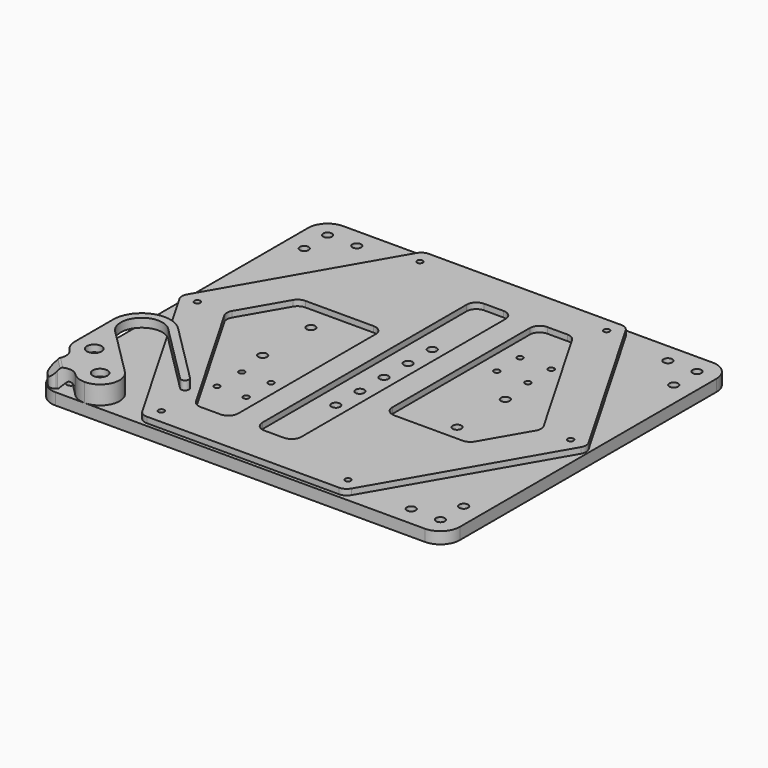
from build123d import *

# Parameters (mm, degrees)
F0_W          = 210
F0_H          = 185
F0_R          = 2
F1_DEPTH      = 6
F2_R          = 10
F3_R          = 1.5
F4_DEPTH      = 6.001
F5_R          = 2.25
F6_DEPTH      = 6.001
F7_R          = 2.25
F8_DEPTH      = 6.001
F9_R          = 2.25
F10_DEPTH     = 6.001
F11_R         = 1.5
F12_DEPTH     = 3
F13_W         = 12.5
F13_H         = 141.2768775266
F14_DEPTH     = 3
F16_DEPTH     = 3
F17_R         = 5
F18_R         = 1.5
F19_DEPTH     = 5
F20_R         = 1.5
F21_DEPTH     = 4.5
F22_R         = 3.75
F23_DEPTH     = 3.5
F24_SIZE      = 2.24999
F26_DEPTH     = 9.5
F28_DEPTH     = 9.5
F29_SIZE      = 5
F31_DEPTH     = 8
F32_T4_DEPTH  = 19.75
F32_T11_DEPTH = 19.75
F33_R         = 3
F34_R         = 1.5


# Not quite as in the source:
# - a fillet or chamfer that OpenCascade refuses, or shapes differently, is made with other operations: its cross-section is extruded or revolved along the edge and cut away or added
# - a fillet or chamfer is up to 0.001 mm smaller than in the source, because OpenCascade refuses the exact size


with BuildPart() as f1:
    # F0 (on Top) → F1 (new body)
    with BuildSketch(Plane.XY):
        Rectangle(F0_W, F0_H)
        with Locations((-48, -83.1384387633)):
            Circle(F0_R, mode=Mode.SUBTRACT)
        with Locations((48, -83.1384387633)):
            Circle(F0_R, mode=Mode.SUBTRACT)
        with Locations((-96, 0)):
            Circle(F0_R, mode=Mode.SUBTRACT)
        with Locations((-48, 83.1384387633)):
            Circle(F0_R, mode=Mode.SUBTRACT)
        with Locations((96, 0)):
            Circle(F0_R, mode=Mode.SUBTRACT)
        with Locations((48, 83.1384387633)):
            Circle(F0_R, mode=Mode.SUBTRACT)
    extrude(amount=F1_DEPTH)

    # F2
    f2_edges = [f1.edges().sort_by_distance(p)[0] for p in [
        (-105, -92.5, 3),
        (105, -92.5, 3),
        (-105, 92.5, 3),
        (105, 92.5, 3),
    ]]
    fillet(f2_edges, radius=F2_R)

    # F3 (on face) → F4 (cut, through all)
    with BuildSketch(Plane(origin=(0, 0, 0), x_dir=(1, 0, 0), z_dir=(0, 0, -1))):
        with Locations((-47.5, 48)):
            Circle(F3_R)
        with Locations((-32.5, 48)):
            Circle(F3_R)
        with Locations((-47.5, 32)):
            Circle(F3_R)
        with Locations((-32.5, 32)):
            Circle(F3_R)
        with Locations((32, -47.5)):
            Circle(F3_R)
        with Locations((32, -32.5)):
            Circle(F3_R)
        with Locations((48, -32.5)):
            Circle(F3_R)
        with Locations((48, -47.5)):
            Circle(F3_R)
    extrude(amount=-F4_DEPTH, mode=Mode.SUBTRACT)

    # F5 (on face) → F6 (cut, through all)
    with BuildSketch(Plane(origin=(0, 0, 0), x_dir=(1, 0, 0), z_dir=(0, 0, -1))):
        with Locations((0, -31)):
            Circle(F5_R)
        Circle(F5_R)
        with Locations((0, 31)):
            Circle(F5_R)
        with Locations((0, -15.5)):
            Circle(F5_R)
        with Locations((0, 15.5)):
            Circle(F5_R)
    extrude(amount=-F6_DEPTH, mode=Mode.SUBTRACT)

    # F7 (on face) → F8 (cut, through all)
    with BuildSketch(Plane(origin=(0, 0, 0), x_dir=(1, 0, 0), z_dir=(0, 0, -1))):
        with Locations((50, 15.5)):
            Circle(F7_R)
        with Locations((50, -15.5)):
            Circle(F7_R)
        with Locations((-50, 15.5)):
            Circle(F7_R)
        with Locations((-50, -15.5)):
            Circle(F7_R)
    extrude(amount=-F8_DEPTH, mode=Mode.SUBTRACT)

    # F9 (on face) → F10 (cut, through all)
    with BuildSketch(Plane(origin=(0, 0, 0), x_dir=(1, 0, 0), z_dir=(0, 0, -1))):
        with Locations((95, 82.5)):
            Circle(F9_R)
        with Locations((95, 67.5)):
            Circle(F9_R)
        with Locations((80, 82.5)):
            Circle(F9_R)
        with Locations((-95, 67.5)):
            Circle(F9_R)
        with Locations((-95, 82.5)):
            Circle(F9_R)
        with Locations((-80, 82.5)):
            Circle(F9_R)
        with Locations((95, -67.5)):
            Circle(F9_R)
        with Locations((95, -82.5)):
            Circle(F9_R)
        with Locations((80, -82.5)):
            Circle(F9_R)
        with Locations((-95, -67.5)):
            Circle(F9_R)
        with Locations((-95, -82.5)):
            Circle(F9_R)
        with Locations((-80, -82.5)):
            Circle(F9_R)
    extrude(amount=-F10_DEPTH, mode=Mode.SUBTRACT)


with BuildPart() as f12:
    # F11 (on face) → F12 (new body)
    with BuildSketch(Plane.XY.offset(6)):
        Polygon((52.3301270189, -90.6384387633), (104.6602540378, 0), (52.3301270189, 90.6384387633), (-52.3301270189, 90.6384387633), (-104.6602540378, 0), (-52.3301270189, -90.6384387633), align=None)
        with Locations((-48, -83.1384387633)):
            Circle(F11_R, mode=Mode.SUBTRACT)
        with Locations((48, -83.1384387633)):
            Circle(F11_R, mode=Mode.SUBTRACT)
        with Locations((-96, 0)):
            Circle(F11_R, mode=Mode.SUBTRACT)
        with Locations((-48, 83.1384387633)):
            Circle(F11_R, mode=Mode.SUBTRACT)
        Polygon((40.7831216351, 70.6384387633), (81.5662432703, 0), (40.7831216351, -70.6384387633), (-40.7831216351, -70.6384387633), (-81.5662432703, 0), (-40.7831216351, 70.6384387633), align=None, mode=Mode.SUBTRACT)
        with Locations((96, 0)):
            Circle(F11_R, mode=Mode.SUBTRACT)
        with Locations((48, 83.1384387633)):
            Circle(F11_R, mode=Mode.SUBTRACT)
    extrude(amount=F12_DEPTH)

    # F13 (on face) → F14 (join, through all)
    with BuildSketch(Plane.XY.offset(9)):
        with Locations((-16.25, 0)):
            Rectangle(F13_W, F13_H)
        with Locations((16.25, 0)):
            Rectangle(F13_W, F13_H)
    extrude(amount=-F14_DEPTH)

    # F15 (on face) → F16 (join, through all)
    with BuildSketch(Plane.XY.offset(9)):
        Polygon((-22.5, 70.6384387633), (-40.7831216351, 70.6384387633), (-65.5447733002, 27.75), (-22.5, 27.75), align=None)
        Polygon((22.5, -27.75), (22.5, -70.6384387633), (40.7831216351, -70.6384387633), (65.5447733002, -27.75), align=None)
    extrude(amount=-F16_DEPTH)

    # F17
    f17_edges = [f12.edges().sort_by_distance(p)[0] for p in [
        (-52.330127, 90.638439, 7.5),
        (-104.660254, 0, 7.5),
        (-52.330127, -90.638439, 7.5),
        (52.330127, -90.638439, 7.5),
        (104.660254, 0, 7.5),
        (52.330127, 90.638439, 7.5),
        (-81.566243, 0, 7.5),
        (-40.783122, -70.638439, 7.5),
        (-22.5, -70.638439, 7.5),
        (-65.544773, 27.75, 7.5),
        (-22.5, 27.75, 7.5),
        (-10, 70.638439, 7.5),
        (10, 70.638439, 7.5),
        (10, -70.638439, 7.5),
        (-10, -70.638439, 7.5),
        (22.5, -27.75, 7.5),
        (65.544773, -27.75, 7.5),
        (81.566243, 0, 7.5),
        (40.783122, 70.638439, 7.5),
        (22.5, 70.638439, 7.5),
    ]]
    fillet(f17_edges, radius=F17_R)


with BuildPart() as f19:
    # F18 (on face) → F19 (new body)
    with BuildSketch(Plane.XY.offset(6)):
        with BuildLine():
            Line((-105, -67.5), (-105, -82.5))
            ThreePointArc((-105, -82.5), (-102.0710678119, -89.5710678119), (-95, -92.5))
            Line((-95, -92.5), (-80, -92.5))
            ThreePointArc((-80, -92.5), (-70.7612046749, -86.3268343237), (-72.9289321881, -75.4289321881))
            Line((-72.9289321881, -75.4289321881), (-87.9289321881, -60.4289321881))
            ThreePointArc((-87.9289321881, -60.4289321881), (-98.8268343237, -58.2612046749), (-105, -67.5))
        make_face()
        with Locations((-95, -82.5)):
            Circle(F18_R, mode=Mode.SUBTRACT)
        with Locations((-80, -82.5)):
            Circle(F18_R, mode=Mode.SUBTRACT)
        with Locations((-95, -67.5)):
            Circle(F18_R, mode=Mode.SUBTRACT)
    extrude(amount=F19_DEPTH)

    # F20 (on face) → F21 (join)
    with BuildSketch(Plane.XY.offset(11)):
        with BuildLine():
            Line((-72.9289321881, -75.4289321881), (-87.9289321881, -60.4289321881))
            Line((-87.9289321881, -60.4289321881), (-97.8653320081, -50.4925323681))
            ThreePointArc((-97.8653320081, -50.4925323681), (-97.8653320081, -35.3570164091), (-82.7298160491, -35.3570164091))
            Line((-82.7298160491, -35.3570164091), (-51.9723484172, -66.1144840409))
            ThreePointArc((-51.9723484172, -66.1144840409), (-49.1439212925, -66.1144840409), (-49.1439212925, -63.2860569162))
            Line((-49.1439212925, -63.2860569162), (-79.9013889243, -32.5285892843))
            ThreePointArc((-79.9013889243, -32.5285892843), (-95.9239488634, -29.3415039554), (-105, -42.9247743886))
            Line((-105, -42.9247743886), (-105, -67.5))
            Line((-105, -67.5), (-105, -82.5))
            ThreePointArc((-105, -82.5), (-102.0710678119, -89.5710678119), (-95, -92.5))
            Line((-95, -92.5), (-80, -92.5))
            ThreePointArc((-80, -92.5), (-70.7612046749, -86.3268343237), (-72.9289321881, -75.4289321881))
        make_face()
        with Locations((-95, -82.5)):
            Circle(F20_R, mode=Mode.SUBTRACT)
        with Locations((-80, -82.5)):
            Circle(F20_R, mode=Mode.SUBTRACT)
        with Locations((-95, -67.5)):
            Circle(F20_R, mode=Mode.SUBTRACT)
    extrude(amount=F21_DEPTH)

    # F22 (on face) → F23 (cut)
    with BuildSketch(Plane.XY.offset(15.5)):
        with Locations((-95, -67.5)):
            Circle(F22_R)
        with Locations((-80, -82.5)):
            Circle(F22_R)
    extrude(amount=-F23_DEPTH, mode=Mode.SUBTRACT)

    # F24 (size 2.25 in the source; OpenCascade refuses exactly that, so slightly less here)
    f24_edges = [f19.edges().sort_by_distance(p)[0] for p in [
        (-96.5, -67.5, 12),
        (-81.5, -82.5, 12),
    ]]
    chamfer(f24_edges, length=F24_SIZE)

    # F25 (on face) → F26 (cut, through all)
    with BuildSketch(Plane.XY.offset(15.5)):
        with BuildLine():
            ThreePointArc((-102.0710678119, -74.5710678119), (-104.2387953251, -71.3268343237), (-105, -67.5))
            Line((-105, -67.5), (-105, -82.5))
            ThreePointArc((-105, -82.5), (-102.0710678119, -89.5710678119), (-95, -92.5))
            Line((-95, -92.5), (-80, -92.5))
            ThreePointArc((-80, -92.5), (-83.8268343237, -91.7387953251), (-87.0710678119, -89.5710678119))
            Line((-87.0710678119, -89.5710678119), (-102.0710678119, -74.5710678119))
        make_face()
    extrude(amount=-F26_DEPTH, mode=Mode.SUBTRACT)

    # F27 (on face) → F28 (join, through all)
    with BuildSketch(Plane.XY.offset(15.5)):
        Polygon((-89.6213203436, -82.7781745931), (-95.2781745931, -77.1213203436), (-104.4705627485, -86.313708499), (-98.813708499, -91.9705627485), align=None)
    extrude(amount=-F28_DEPTH)

    # F29
    f29_edges = [f19.edges().sort_by_distance(p)[0] for p in [
        (-101.642136, -89.142136, 15.5),
    ]]
    chamfer(f29_edges, length=F29_SIZE)

    # F30 (on face) → F31 (cut, through all)
    with BuildSketch(Plane(origin=(-3.4215728753, 3.4215728753, 0), x_dir=(0.7071067812, 0.7071067812, 0), z_dir=(0.7071067812, -0.7071067812, 0))):
        Polygon((-124.9048519428, 6), (-124.9048519428, 12), (-130.9048519428, 6), align=None)
    extrude(amount=-F31_DEPTH, mode=Mode.SUBTRACT)

    # F32: fillet of radius 6.5 on 2 edges, made by hand


with BuildPart() as f32_tool2:
    # F32_s3 → F32_t4 (new body)
    with BuildSketch(Plane.XY.offset(15.5)):
        with BuildLine():
            ThreePointArc((-96.3388347648, -89.4956890143), (-91.7426406871, -87.591883092), (-87.1464466094, -89.4956890143))
            Line((-87.1464466094, -89.4956890143), (-91.7426406871, -84.8994949366))
            Line((-91.7426406871, -84.8994949366), (-96.3388347648, -89.4956890143))
        make_face()
    extrude(amount=-F32_T4_DEPTH)

    split(bisect_by=Plane.XY.offset(6), keep=Keep.TOP)

    split(bisect_by=Plane(origin=(-48.4031745931, -48.4031745931, 68.4524259714), x_dir=(0.7071067812, -0.7071067812, 0), z_dir=(-0.5, -0.5, 0.7071067812)), keep=Keep.TOP)

    split(bisect_by=Plane(origin=(-51.4083784131, -51.4083784131, 72.7024259714), x_dir=(-0.7071067812, 0.7071067812, 0), z_dir=(0.5, 0.5, -0.7071067812)), keep=Keep.TOP)


with BuildPart() as f19_1:
    add(f19.part)

    # F32_t1: union F32_tool2
    add(f32_tool2.part)


with BuildPart() as f32_tool9:
    # F32_s10 → F32_t11 (new body)
    with BuildSketch(Plane.XY.offset(-4.25)):
        with BuildLine():
            ThreePointArc((-101.9956890143, -74.6464466094), (-100.091883092, -79.2426406871), (-101.9956890143, -83.8388347648))
            Line((-101.9956890143, -83.8388347648), (-97.3994949366, -79.2426406871))
            Line((-97.3994949366, -79.2426406871), (-101.9956890143, -74.6464466094))
        make_face()
    extrude(amount=F32_T11_DEPTH)

    split(bisect_by=Plane.XY.offset(6), keep=Keep.TOP)

    split(bisect_by=Plane(origin=(-48.4031745931, -48.4031745931, 68.4524259714), x_dir=(0.7071067812, -0.7071067812, 0), z_dir=(-0.5, -0.5, 0.7071067812)), keep=Keep.TOP)

    split(bisect_by=Plane(origin=(-51.4083784131, -51.4083784131, 72.7024259714), x_dir=(-0.7071067812, 0.7071067812, 0), z_dir=(0.5, 0.5, -0.7071067812)), keep=Keep.TOP)


with BuildPart() as f19_2:
    add(f19_1.part)

    # F32_t8: union F32_tool9
    add(f32_tool9.part)

    # F33
    f33_edges = [f19_2.edges().sort_by_distance(p)[0] for p in [
        (-98.813708, -91.970563, 8.25),
        (-104.470563, -86.313708, 8.25),
    ]]
    fillet(f33_edges, radius=F33_R)

    # F34
    f34_edges = [f19_2.edges().sort_by_distance(p)[0] for p in [
        (-94.571068, -82.071068, 12),
        (-98.106602, -85.606602, 15.5),
    ]]
    fillet(f34_edges, radius=F34_R)


solid = Compound([f1.part, f12.part, f19_2.part])
